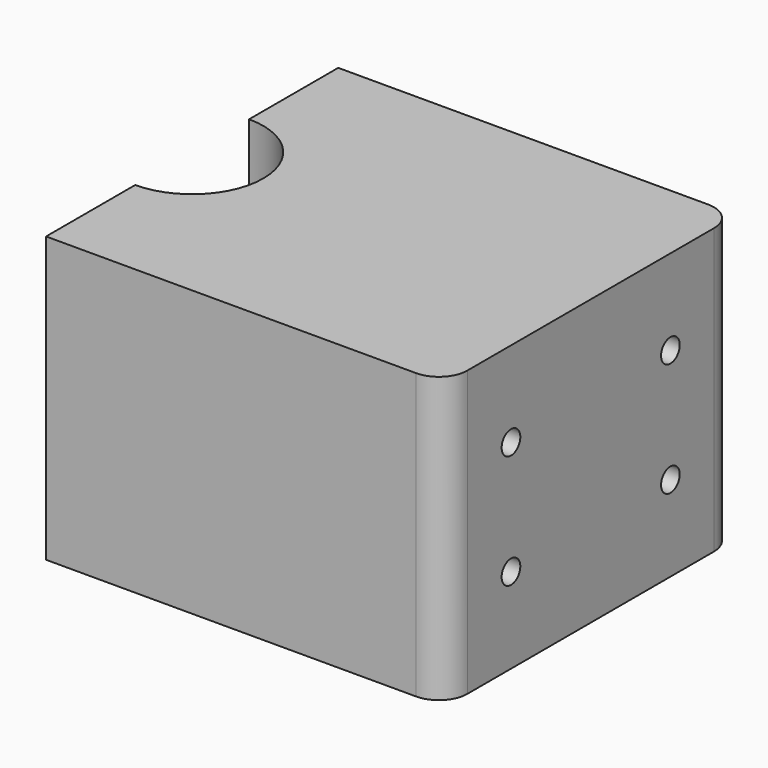
from build123d import *

# Parameters (mm, degrees)
F1_DEPTH = 25.4
F3_D     = 2.0828


# Not quite as in the source:
# - a feature names something its author has since deleted; it is built from what else it names


with BuildPart() as f1:
    # F0 (on Top) → F1 (new body)
    with BuildSketch(Plane.XY):
        with BuildLine():
            Line((-17.78, -6.35), (-17.78, -16.29156))
            Line((-17.78, -16.29156), (15.24, -16.29156))
            ThreePointArc((15.24, -16.29156), (17.0360512242, -15.5476112242), (17.78, -13.75156))
            Line((17.78, -13.75156), (17.78, 13.75156))
            ThreePointArc((17.78, 13.75156), (17.0360512242, 15.5476112242), (15.24, 16.29156))
            Line((15.24, 16.29156), (-17.78, 16.29156))
            Line((-17.78, 16.29156), (-17.78, 6.35))
            ThreePointArc((-17.78, 6.35), (-11.43, 0), (-17.78, -6.35))
        make_face()
    extrude(amount=F1_DEPTH)

    # F3 (through all)
    with Locations(Plane.YZ.offset(17.78)):
        with Locations((-8.89, 17.78), (-8.89, 7.62), (8.89, 17.78), (8.89, 7.62)):
            Hole(F3_D / 2)


solid = f1.part
